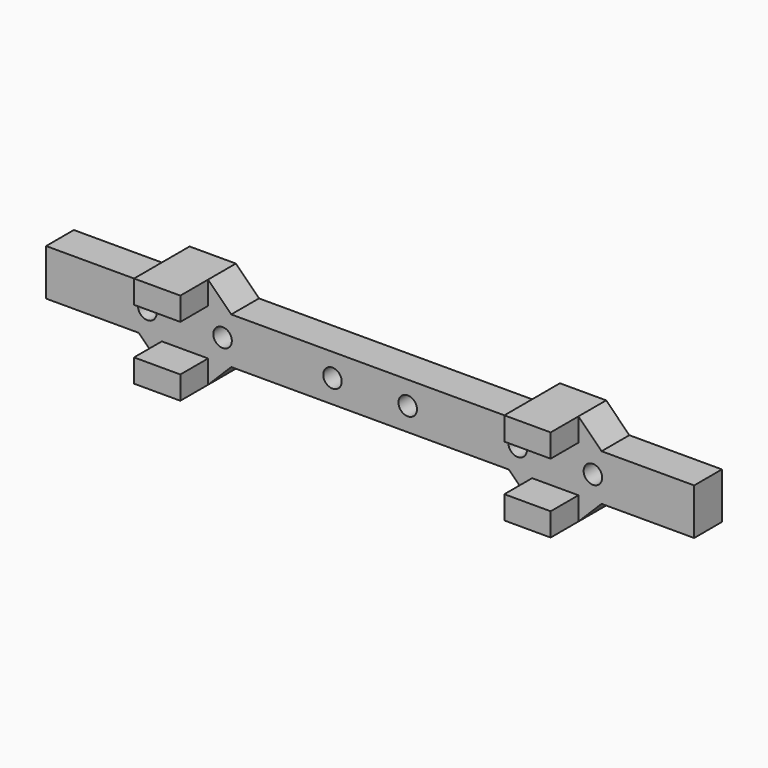
from build123d import *

# Parameters (mm, degrees)
F0_W     = 50
F0_H     = 20
F0_R     = 4
F0_W_2   = 20
F0_W_3   = 140
F1_DEPTH = 15
F0_H_2   = 10
F2_DEPTH = 30
F3_SIZE  = 9.99999


# Not quite as in the source:
# - a fillet or chamfer is up to 0.001 mm smaller than in the source, because OpenCascade refuses the exact size
# - a feature names something its author has since deleted; it is built from what else it names


with BuildPart() as f1:
    # F0 (on Front) → F1 (new body)
    with BuildSketch(Plane.XZ):
        with Locations((-115, 10)):
            Rectangle(F0_W, F0_H)
        with Locations((-96.25, 10)):
            Circle(F0_R, mode=Mode.SUBTRACT)
        with Locations((-80, 10)):
            Rectangle(F0_W_2, F0_H)
        with Locations((80, 10)):
            Rectangle(F0_W_2, F0_H)
        with Locations((115, 10)):
            Rectangle(F0_W, F0_H)
        with Locations((96.25, 10)):
            Circle(F0_R, mode=Mode.SUBTRACT)
        with Locations((0, 10)):
            Rectangle(F0_W_3, F0_H)
        with Locations((-63.75, 10)):
            Circle(F0_R, mode=Mode.SUBTRACT)
        with Locations((-16.25, 10)):
            Circle(F0_R, mode=Mode.SUBTRACT)
        with Locations((16.25, 10)):
            Circle(F0_R, mode=Mode.SUBTRACT)
        with Locations((63.75, 10)):
            Circle(F0_R, mode=Mode.SUBTRACT)
    extrude(amount=F1_DEPTH)

    # F0 (on Front) → F2 (join)
    with BuildSketch(Plane.XZ):
        with Locations((80, 25)):
            Rectangle(F0_W_2, F0_H_2)
        with Locations((-80, 25)):
            Rectangle(F0_W_2, F0_H_2)
        with Locations((-80, -5)):
            Rectangle(F0_W_2, F0_H_2)
        with Locations((80, -5)):
            Rectangle(F0_W_2, F0_H_2)
    extrude(amount=F2_DEPTH)

    # F3 (size 10 in the source; OpenCascade refuses exactly that, so slightly less here)
    f3_edges = [f1.edges().sort_by_distance(p)[0] for p in [
        (70, -7.5, 20),
        (90, -7.5, 20),
        (-70, -7.5, 20),
        (-90, -7.5, 20),
        (-90, -7.5, 0),
        (-70, -7.5, 0),
        (70, -7.5, 0),
        (90, -7.5, 0),
    ]]
    chamfer(f3_edges, length=F3_SIZE)


solid = f1.part
